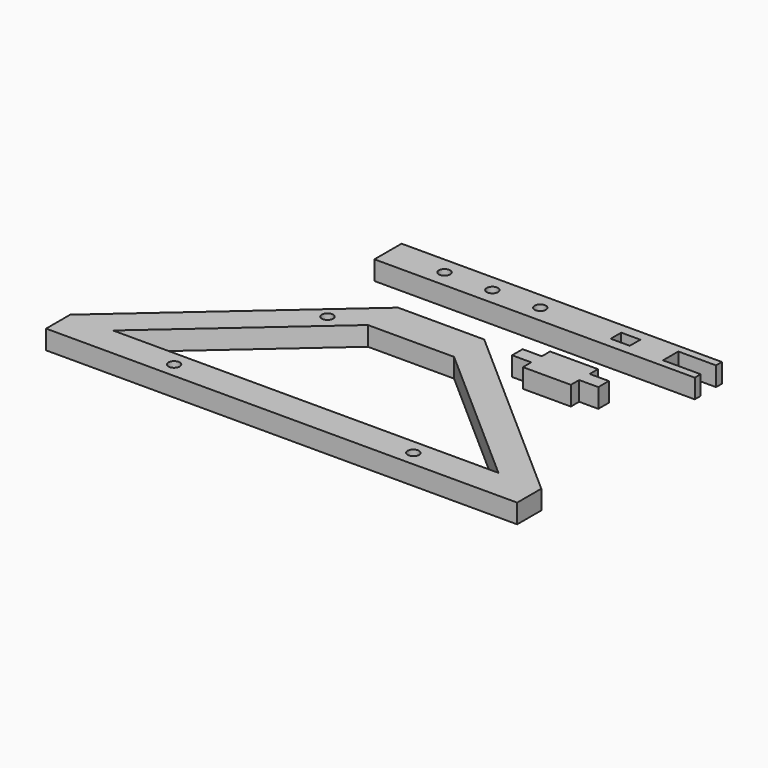
from build123d import *

# Parameters (mm, degrees)
F0_R     = 1.5
F0_W     = 5.08
F0_H     = 3.5
F1_DEPTH = 5.08
F0_W_2   = 11.4325
F0_H_2   = 10


# Not quite as in the source:
# - a feature names something its author has since deleted; it is built from what else it names


with BuildPart() as f1:
    # F0 (on Top) → F1 (new body)
    with BuildSketch(Plane.XY):
        Polygon((4.9954398084, 48.7905830651), (4.9954398084, 50.7505830651), (-80.0045601916, 50.7505830651), (-80.0045601916, 41.7505830651), (4.9954398084, 41.7505830651), (4.9954398084, 43.7105830651), (-5.0045601916, 43.7105830651), (-5.0045601916, 48.7905830651), align=None)
        with Locations((-65.0045601916, 46.2505830651)):
            Circle(F0_R, mode=Mode.SUBTRACT)
        with Locations((-52.3045601916, 46.2505830651)):
            Circle(F0_R, mode=Mode.SUBTRACT)
        with Locations((-39.6045601916, 46.2505830651)):
            Circle(F0_R, mode=Mode.SUBTRACT)
        with Locations((-16.9845601916, 46.2505830651)):
            Rectangle(F0_W, F0_H, mode=Mode.SUBTRACT)
    extrude(amount=F1_DEPTH)


with BuildPart() as f1b:
    # F0 (on Top) → F1, piece 2 (new body)
    with BuildSketch(Plane.XY):
        Polygon((-19.3953289995, 32.1917034835), (-25.7478289995, 32.1917034835), (-25.7478289995, 29.4417034835), (-25.7478289995, 25.9417034835), (-25.7478289995, 23.1917034835), (-19.3953289995, 23.1917034835), align=None)
        with Locations((-28.2878289995, 27.6917034835)):
            Rectangle(F0_W, F0_H)
        Polygon((-13.0428289995, 32.1917034835), (-19.3953289995, 32.1917034835), (-19.3953289995, 23.1917034835), (-13.0428289995, 23.1917034835), (-13.0428289995, 25.9417034835), (-13.0428289995, 29.4417034835), align=None)
        with Locations((-10.5028289995, 27.6917034835)):
            Rectangle(F0_W, F0_H)
    extrude(amount=F1_DEPTH)


with BuildPart() as f1c:
    # F0 (on Top) → F1, piece 3 (new body)
    with BuildSketch(Plane.XY):
        Polygon((-51.2056094673, 27.870685693), (-62.6381094673, 27.870685693), (-62.6381094673, 22.870685693), (-62.6381094673, 17.870685693), (-51.2056094673, 17.870685693), align=None)
        with Locations((-45.4893594673, 22.870685693)):
            Rectangle(F0_W_2, F0_H_2)
        Polygon((-62.6381094673, 22.870685693), (-62.6381094673, 27.870685693), (-113.7056094673, -17.0304328203), (-102.3322847728, -17.0304328203), (-62.6381094673, 17.870685693), align=None)
        with BuildLine():
            ThreePointArc((-70.0347154799, 15.5836834659), (-72.9472734976, 15.0790253177), (-70.3742886087, 16.5341620173))
            ThreePointArc((-70.3742886087, 16.5341620173), (-70.1221574622, 16.0883416142), (-70.0347154799, 15.5836834659))
        make_face(mode=Mode.SUBTRACT)
        Polygon((11.2943905327, -17.0304328203), (-39.7731094673, 27.870685693), (-39.7731094673, 17.870685693), (-0.0789341619, -17.0304328203), align=None)
        Polygon((-102.3322847728, -17.0304328203), (-113.7056094673, -17.0304328203), (-113.7056094673, -25.0304328203), (-51.2056094673, -25.0304328203), (-51.2056094673, -17.0304328203), align=None)
        with Locations((-82.9556094673, -21.0304328203)):
            Circle(F0_R, mode=Mode.SUBTRACT)
        Polygon((11.2943905327, -25.0304328203), (11.2943905327, -17.0304328203), (-0.0789341619, -17.0304328203), (-51.2056094673, -17.0304328203), (-51.2056094673, -25.0304328203), align=None)
        with Locations((-19.4556094673, -21.0304328203)):
            Circle(F0_R, mode=Mode.SUBTRACT)
    extrude(amount=F1_DEPTH)


solid = Compound([f1.part, f1b.part, f1c.part])
